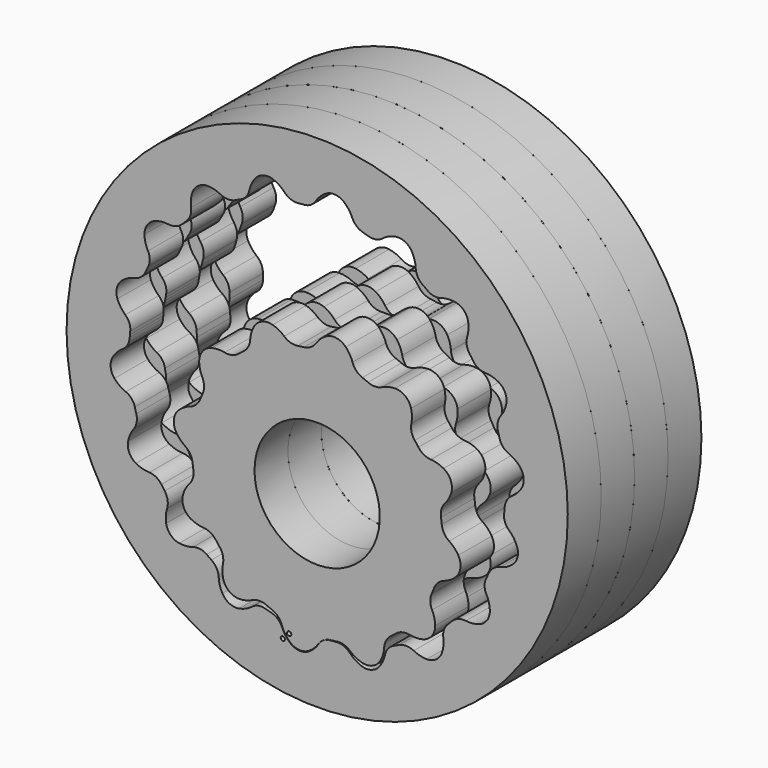
from build123d import *

# Parameters (mm, degrees)
F0_R      = 9.525
F0_R_2    = 0.3175
F1_DEPTH  = 6.35
F0_R_3    = 38.1
F2_DEPTH  = 6.35
F3_R      = 2.54
F4_R      = 2.4892
F5_R      = 2.54
F6_R      = 2.286
F7_R      = 2.413
F9_ANGLE  = 0.02
F11_ANGLE = 7.5
F12_ANGLE = 4.9999
F14_ANGLE = 180
F15_ANGLE = 7.5
F16_ANGLE = 4.9999


with BuildPart() as f1:
    # F0 (on Front) → F1 (new body)
    with BuildSketch(Plane.XZ):
        with BuildLine():
            ThreePointArc((18.7854166667, -3.1639564883), (18.9837389297, -1.5875), (19.05, 0))
            ThreePointArc((19.05, 0), (18.9837389297, 1.5875), (18.7854166667, 3.1639564883))
            ThreePointArc((18.7854166667, 3.1639564883), (18.4008869908, 4.9305028092), (17.8506262981, 6.652641638))
            ThreePointArc((17.8506262981, 6.652641638), (16.4977839421, 9.525), (14.6866698099, 12.1327750287))
            ThreePointArc((14.6866698099, 12.1327750287), (13.4703841816, 13.4703841816), (12.1327750287, 14.6866698099))
            ThreePointArc((12.1327750287, 14.6866698099), (9.525, 16.4977839421), (6.652641638, 17.8506262981))
            ThreePointArc((6.652641638, 17.8506262981), (4.9305028092, 18.4008869908), (3.1639564883, 18.7854166667))
            ThreePointArc((3.1639564883, 18.7854166667), (0, 19.05), (-3.1639564883, 18.7854166667))
            ThreePointArc((-3.1639564883, 18.7854166667), (-4.9305028092, 18.4008869908), (-6.652641638, 17.8506262981))
            ThreePointArc((-6.652641638, 17.8506262981), (-9.525, 16.4977839421), (-12.1327750287, 14.6866698099))
            ThreePointArc((-12.1327750287, 14.6866698099), (-13.4703841816, 13.4703841816), (-14.6866698099, 12.1327750287))
            ThreePointArc((-14.6866698099, 12.1327750287), (-16.4977839421, 9.525), (-17.8506262981, 6.652641638))
            ThreePointArc((-17.8506262981, 6.652641638), (-18.4008869908, 4.9305028092), (-18.7854166667, 3.1639564883))
            ThreePointArc((-18.7854166667, 3.1639564883), (-19.05, 0), (-18.7854166667, -3.1639564883))
            ThreePointArc((-18.7854166667, -3.1639564883), (-18.4008869908, -4.9305028092), (-17.8506262981, -6.652641638))
            ThreePointArc((-17.8506262981, -6.652641638), (-16.4977839421, -9.525), (-14.6866698099, -12.1327750287))
            ThreePointArc((-14.6866698099, -12.1327750287), (-13.4703841816, -13.4703841816), (-12.1327750287, -14.6866698099))
            ThreePointArc((-12.1327750287, -14.6866698099), (-9.525, -16.4977839421), (-6.652641638, -17.8506262981))
            ThreePointArc((-6.652641638, -17.8506262981), (-4.9305028092, -18.4008869908), (-3.1639564883, -18.7854166667))
            ThreePointArc((-3.1639564883, -18.7854166667), (0, -19.05), (3.1639564883, -18.7854166667))
            ThreePointArc((3.1639564883, -18.7854166667), (4.9305028092, -18.4008869908), (6.652641638, -17.8506262981))
            ThreePointArc((6.652641638, -17.8506262981), (9.525, -16.4977839421), (12.1327750287, -14.6866698099))
            ThreePointArc((12.1327750287, -14.6866698099), (13.4703841816, -13.4703841816), (14.6866698099, -12.1327750287))
            ThreePointArc((14.6866698099, -12.1327750287), (16.4977839421, -9.525), (17.8506262981, -6.652641638))
            ThreePointArc((17.8506262981, -6.652641638), (18.4008869908, -4.9305028092), (18.7854166667, -3.1639564883))
        make_face()
        Circle(F0_R, mode=Mode.SUBTRACT)
        with BuildLine():
            ThreePointArc((-3.1639564883, 18.7854166667), (0, 19.05), (3.1639564883, 18.7854166667))
            ThreePointArc((3.1639564883, 18.7854166667), (2.0640323089, 20.9486335794), (0, 22.225))
            ThreePointArc((0, 22.225), (-2.0640323089, 20.9486335794), (-3.1639564883, 18.7854166667))
        make_face()
        with BuildLine():
            ThreePointArc((-12.1327750287, 14.6866698099), (-9.525, 16.4977839421), (-6.652641638, 17.8506262981))
            ThreePointArc((-6.652641638, 17.8506262981), (-8.686812376, 19.1740650088), (-11.1125, 19.2474145991))
            ThreePointArc((-11.1125, 19.2474145991), (-12.2618212034, 17.1100326999), (-12.1327750287, 14.6866698099))
        make_face()
        with BuildLine():
            ThreePointArc((-17.8506262981, 6.652641638), (-16.4977839421, 9.525), (-14.6866698099, 12.1327750287))
            ThreePointArc((-14.6866698099, 12.1327750287), (-17.1100326999, 12.2618212034), (-19.2474145991, 11.1125))
            ThreePointArc((-19.2474145991, 11.1125), (-19.1740650088, 8.686812376), (-17.8506262981, 6.652641638))
        make_face()
        with BuildLine():
            ThreePointArc((-18.7854166667, -3.1639564883), (-19.05, 0), (-18.7854166667, 3.1639564883))
            ThreePointArc((-18.7854166667, 3.1639564883), (-20.9486335794, 2.0640323089), (-22.225, 0))
            ThreePointArc((-22.225, 0), (-20.9486335794, -2.0640323089), (-18.7854166667, -3.1639564883))
        make_face()
        with BuildLine():
            ThreePointArc((-19.2474145991, -11.1125), (-17.1100326999, -12.2618212034), (-14.6866698099, -12.1327750287))
            ThreePointArc((-14.6866698099, -12.1327750287), (-16.4977839421, -9.525), (-17.8506262981, -6.652641638))
            ThreePointArc((-17.8506262981, -6.652641638), (-19.1740650088, -8.686812376), (-19.2474145991, -11.1125))
        make_face()
        with BuildLine():
            ThreePointArc((6.652641638, 17.8506262981), (9.525, 16.4977839421), (12.1327750287, 14.6866698099))
            ThreePointArc((12.1327750287, 14.6866698099), (12.2618212034, 17.1100326999), (11.1125, 19.2474145991))
            ThreePointArc((11.1125, 19.2474145991), (8.686812376, 19.1740650088), (6.652641638, 17.8506262981))
        make_face()
        with BuildLine():
            ThreePointArc((14.6866698099, 12.1327750287), (16.4977839421, 9.525), (17.8506262981, 6.652641638))
            ThreePointArc((17.8506262981, 6.652641638), (19.1740650088, 8.686812376), (19.2474145991, 11.1125))
            ThreePointArc((19.2474145991, 11.1125), (17.1100326999, 12.2618212034), (14.6866698099, 12.1327750287))
        make_face()
        with BuildLine():
            ThreePointArc((18.7854166667, 3.1639564883), (18.9837389297, 1.5875), (19.05, 0))
            ThreePointArc((19.05, 0), (18.9837389297, -1.5875), (18.7854166667, -3.1639564883))
            ThreePointArc((18.7854166667, -3.1639564883), (20.9486335794, -2.0640323089), (22.225, 0))
            ThreePointArc((22.225, 0), (20.9486335794, 2.0640323089), (18.7854166667, 3.1639564883))
        make_face()
        with BuildLine():
            ThreePointArc((19.2474145991, -11.1125), (19.1740650088, -8.686812376), (17.8506262981, -6.652641638))
            ThreePointArc((17.8506262981, -6.652641638), (16.4977839421, -9.525), (14.6866698099, -12.1327750287))
            ThreePointArc((14.6866698099, -12.1327750287), (17.1100326999, -12.2618212034), (19.2474145991, -11.1125))
        make_face()
        with BuildLine():
            ThreePointArc((-11.1125, -19.2474145991), (-8.686812376, -19.1740650088), (-6.652641638, -17.8506262981))
            ThreePointArc((-6.652641638, -17.8506262981), (-9.525, -16.4977839421), (-12.1327750287, -14.6866698099))
            ThreePointArc((-12.1327750287, -14.6866698099), (-12.2618212034, -17.1100326999), (-11.1125, -19.2474145991))
        make_face()
        with BuildLine():
            ThreePointArc((0, -22.225), (2.0640323089, -20.9486335794), (3.1639564883, -18.7854166667))
            ThreePointArc((3.1639564883, -18.7854166667), (0, -19.05), (-3.1639564883, -18.7854166667))
            ThreePointArc((-3.1639564883, -18.7854166667), (-2.0640323089, -20.9486335794), (0, -22.225))
        make_face()
        with Locations((1.5819782441, -20.5052083333)):
            Circle(F0_R_2, mode=Mode.SUBTRACT)
        with BuildLine():
            ThreePointArc((11.1125, -19.2474145991), (12.2618212034, -17.1100326999), (12.1327750287, -14.6866698099))
            ThreePointArc((12.1327750287, -14.6866698099), (9.525, -16.4977839421), (6.652641638, -17.8506262981))
            ThreePointArc((6.652641638, -17.8506262981), (8.686812376, -19.1740650088), (11.1125, -19.2474145991))
        make_face()
    extrude(amount=-F1_DEPTH)

    # F3
    f3_edges = [f1.edges().sort_by_distance(p)[0] for p in [
        (-3.163956, 3.175, -18.785417),
        (3.163956, 3.175, -18.785417),
        (6.652642, 3.175, -17.850626),
        (-6.652642, 3.175, -17.850626),
        (-12.132775, 3.175, -14.68667),
        (-14.68667, 3.175, -12.132775),
        (12.132775, 3.175, -14.68667),
        (14.68667, 3.175, -12.132775),
        (17.850626, 3.175, -6.652642),
        (-17.850626, 3.175, -6.652642),
        (-18.785417, 3.175, -3.163956),
        (-18.785417, 3.175, 3.163956),
        (-17.850626, 3.175, 6.652642),
        (-14.68667, 3.175, 12.132775),
        (-12.132775, 3.175, 14.68667),
        (-6.652642, 3.175, 17.850626),
        (-3.163956, 3.175, 18.785417),
        (3.163956, 3.175, 18.785417),
        (6.652642, 3.175, 17.850626),
        (12.132775, 3.175, 14.68667),
        (14.68667, 3.175, 12.132775),
        (17.850626, 3.175, 6.652642),
        (18.785417, 3.175, 3.163956),
        (18.785417, 3.175, -3.163956),
    ]]
    fillet(f3_edges, radius=F3_R)

    # F4
    f4_edges = [f1.edges().sort_by_distance(p)[0] for p in [
        (0, 3.175, -22.225),
        (11.1125, 3.175, -19.247415),
        (-11.1125, 3.175, -19.247415),
        (-19.247415, 3.175, -11.1125),
        (19.247415, 3.175, -11.1125),
        (22.225, 3.175, 0),
        (-22.225, 3.175, 0),
        (-19.247415, 3.175, 11.1125),
        (-11.1125, 3.175, 19.247415),
        (0, 3.175, 22.225),
        (11.1125, 3.175, 19.247415),
        (19.247415, 3.175, 11.1125),
    ]]
    fillet(f4_edges, radius=F4_R)


with BuildPart() as f2:
    # F0 (on Front) → F2 (new body)
    with BuildSketch(Plane.XZ):
        Circle(F0_R_3)
        with Locations((2.5347402211, -30.9479771842)):
            Circle(F0_R_2, mode=Mode.SUBTRACT)
        with BuildLine():
            ThreePointArc((28.517262004, 1.8155970902), (28.5605618534, 0.9082574621), (28.575, 0))
            ThreePointArc((28.575, 0), (28.5605618534, -0.9082574621), (28.517262004, -1.8155970902))
            ThreePointArc((28.517262004, -1.8155970902), (30.3985169788, -3.2859843886), (31.2615712993, -5.5122584794))
            ThreePointArc((31.2615712993, -5.5122584794), (29.6891349394, -7.309089852), (27.4184314472, -8.0473748499))
            ThreePointArc((27.4184314472, -8.0473748499), (26.851716639, -9.7732255955), (26.1764898932, -11.4595812258))
            ThreePointArc((26.1764898932, -11.4595812258), (27.4413892362, -13.484720416), (27.490964429, -15.8719157133))
            ThreePointArc((27.490964429, -15.8719157133), (25.3988050613, -17.0225799857), (23.0125334049, -16.9397146165))
            ThreePointArc((23.0125334049, -16.9397146165), (21.8897199621, -18.3676559468), (20.6784467774, -19.7213707403))
            ThreePointArc((20.6784467774, -19.7213707403), (21.17442496, -22.0570001479), (20.4045415251, -24.3171856677))
            ThreePointArc((20.4045415251, -24.3171856677), (18.0450044464, -24.6828957467), (15.8309842052, -23.7888747968))
            ThreePointArc((15.8309842052, -23.7888747968), (14.2875, -24.7466759131), (12.6862777989, -25.604471887))
            ThreePointArc((12.6862777989, -25.604471887), (12.3535125324, -27.9688801353), (10.8570297743, -29.8294441471))
            ThreePointArc((10.8570297743, -29.8294441471), (8.5147099793, -29.3660899998), (6.7399846698, -27.7687455902))
            ThreePointArc((6.7399846698, -27.7687455902), (4.9619966768, -28.1408815423), (3.1639564883, -28.3992958423))
            ThreePointArc((3.1639564883, -28.3992958423), (2.0425841749, -30.5073004017), (0, -31.7438314267))
            ThreePointArc((0, -31.7438314267), (-2.0425841749, -30.5073004017), (-3.1639564883, -28.3992958423))
            ThreePointArc((-3.1639564883, -28.3992958423), (-4.9619966768, -28.1408815423), (-6.7399846698, -27.7687455902))
            ThreePointArc((-6.7399846698, -27.7687455902), (-8.5147099793, -29.3660899998), (-10.8570297743, -29.8294441471))
            ThreePointArc((-10.8570297743, -29.8294441471), (-12.3535125324, -27.9688801353), (-12.6862777989, -25.604471887))
            ThreePointArc((-12.6862777989, -25.604471887), (-14.2875, -24.7466759131), (-15.8309842052, -23.7888747968))
            ThreePointArc((-15.8309842052, -23.7888747968), (-18.0450044464, -24.6828957467), (-20.4045415251, -24.3171856677))
            ThreePointArc((-20.4045415251, -24.3171856677), (-21.17442496, -22.0570001479), (-20.6784467774, -19.7213707403))
            ThreePointArc((-20.6784467774, -19.7213707403), (-21.8897199621, -18.3676559468), (-23.0125334049, -16.9397146165))
            ThreePointArc((-23.0125334049, -16.9397146165), (-25.3988050613, -17.0225799857), (-27.490964429, -15.8719157133))
            ThreePointArc((-27.490964429, -15.8719157133), (-27.4413892362, -13.484720416), (-26.1764898932, -11.4595812258))
            ThreePointArc((-26.1764898932, -11.4595812258), (-26.851716639, -9.7732255955), (-27.4184314472, -8.0473748499))
            ThreePointArc((-27.4184314472, -8.0473748499), (-29.6891349394, -7.309089852), (-31.2615712993, -5.5122584794))
            ThreePointArc((-31.2615712993, -5.5122584794), (-30.3985169788, -3.2859843886), (-28.517262004, -1.8155970902))
            ThreePointArc((-28.517262004, -1.8155970902), (-28.575, 0), (-28.517262004, 1.8155970902))
            ThreePointArc((-28.517262004, 1.8155970902), (-30.3985169788, 3.2859843886), (-31.2615712993, 5.5122584794))
            ThreePointArc((-31.2615712993, 5.5122584794), (-29.6891349394, 7.309089852), (-27.4184314472, 8.0473748499))
            ThreePointArc((-27.4184314472, 8.0473748499), (-26.851716639, 9.7732255955), (-26.1764898932, 11.4595812258))
            ThreePointArc((-26.1764898932, 11.4595812258), (-27.4413892362, 13.484720416), (-27.490964429, 15.8719157133))
            ThreePointArc((-27.490964429, 15.8719157133), (-25.3988050613, 17.0225799857), (-23.0125334049, 16.9397146165))
            ThreePointArc((-23.0125334049, 16.9397146165), (-21.8897199621, 18.3676559468), (-20.6784467774, 19.7213707403))
            ThreePointArc((-20.6784467774, 19.7213707403), (-21.17442496, 22.0570001479), (-20.4045415251, 24.3171856677))
            ThreePointArc((-20.4045415251, 24.3171856677), (-18.0450044464, 24.6828957467), (-15.8309842052, 23.7888747968))
            ThreePointArc((-15.8309842052, 23.7888747968), (-14.2875, 24.7466759131), (-12.6862777989, 25.604471887))
            ThreePointArc((-12.6862777989, 25.604471887), (-12.3535125324, 27.9688801353), (-10.8570297743, 29.8294441471))
            ThreePointArc((-10.8570297743, 29.8294441471), (-8.5147099793, 29.3660899998), (-6.7399846698, 27.7687455902))
            ThreePointArc((-6.7399846698, 27.7687455902), (-4.9619966768, 28.1408815423), (-3.1639564883, 28.3992958423))
            ThreePointArc((-3.1639564883, 28.3992958423), (-2.0425841749, 30.5073004017), (0, 31.7438314267))
            ThreePointArc((0, 31.7438314267), (2.0425841749, 30.5073004017), (3.1639564883, 28.3992958423))
            ThreePointArc((3.1639564883, 28.3992958423), (4.9619966768, 28.1408815423), (6.7399846698, 27.7687455902))
            ThreePointArc((6.7399846698, 27.7687455902), (8.5147099793, 29.3660899998), (10.8570297743, 29.8294441471))
            ThreePointArc((10.8570297743, 29.8294441471), (12.3535125324, 27.9688801353), (12.6862777989, 25.604471887))
            ThreePointArc((12.6862777989, 25.604471887), (14.2875, 24.7466759131), (15.8309842052, 23.7888747968))
            ThreePointArc((15.8309842052, 23.7888747968), (18.0450044464, 24.6828957467), (20.4045415251, 24.3171856677))
            ThreePointArc((20.4045415251, 24.3171856677), (21.17442496, 22.0570001479), (20.6784467774, 19.7213707403))
            ThreePointArc((20.6784467774, 19.7213707403), (21.8897199621, 18.3676559468), (23.0125334049, 16.9397146165))
            ThreePointArc((23.0125334049, 16.9397146165), (25.3988050613, 17.0225799857), (27.490964429, 15.8719157133))
            ThreePointArc((27.490964429, 15.8719157133), (27.4413892362, 13.484720416), (26.1764898932, 11.4595812258))
            ThreePointArc((26.1764898932, 11.4595812258), (26.851716639, 9.7732255955), (27.4184314472, 8.0473748499))
            ThreePointArc((27.4184314472, 8.0473748499), (29.6891349394, 7.309089852), (31.2615712993, 5.5122584794))
            ThreePointArc((31.2615712993, 5.5122584794), (30.3985169788, 3.2859843886), (28.517262004, 1.8155970902))
        make_face(mode=Mode.SUBTRACT)
    extrude(amount=-F2_DEPTH)

    # F5
    f5_edges = [f2.edges().sort_by_distance(p)[0] for p in [
        (3.163956, 3.175, -28.399296),
        (12.686278, 3.175, -25.604472),
        (20.678447, 3.175, -19.721371),
        (-6.739985, 3.175, -27.768746),
        (-15.830984, 3.175, -23.788875),
        (-23.012533, 3.175, -16.939715),
        (-27.418431, 3.175, -8.047375),
        (26.17649, 3.175, -11.459581),
        (28.517262, 3.175, -1.815597),
        (27.418431, 3.175, 8.047375),
        (23.012533, 3.175, 16.939715),
        (-28.517262, 3.175, 1.815597),
        (-26.17649, 3.175, 11.459581),
        (-20.678447, 3.175, 19.721371),
        (-12.686278, 3.175, 25.604472),
        (-3.163956, 3.175, 28.399296),
        (6.739985, 3.175, 27.768746),
        (15.830984, 3.175, 23.788875),
    ]]
    fillet(f5_edges, radius=F5_R)

    # F6
    f6_edges = [f2.edges().sort_by_distance(p)[0] for p in [
        (-3.163956, 3.175, -28.399296),
        (6.739985, 3.175, -27.768746),
        (-12.686278, 3.175, -25.604472),
        (-20.678447, 3.175, -19.721371),
        (15.830984, 3.175, -23.788875),
        (23.012533, 3.175, -16.939715),
        (-26.17649, 3.175, -11.459581),
        (-28.517262, 3.175, -1.815597),
        (27.418431, 3.175, -8.047375),
        (28.517262, 3.175, 1.815597),
        (26.17649, 3.175, 11.459581),
        (20.678447, 3.175, 19.721371),
        (12.686278, 3.175, 25.604472),
        (3.163956, 3.175, 28.399296),
        (-6.739985, 3.175, 27.768746),
        (-15.830984, 3.175, 23.788875),
        (-23.012533, 3.175, 16.939715),
        (-27.418431, 3.175, 8.047375),
    ]]
    fillet(f6_edges, radius=F6_R)

    # F7
    f7_edges = [f2.edges().sort_by_distance(p)[0] for p in [
        (0, 3.175, -31.743831),
        (10.85703, 3.175, -29.829444),
        (20.404542, 3.175, -24.317186),
        (27.490964, 3.175, -15.871916),
        (-10.85703, 3.175, -29.829444),
        (-20.404542, 3.175, -24.317186),
        (-27.490964, 3.175, -15.871916),
        (-31.261571, 3.175, -5.512258),
        (-31.261571, 3.175, 5.512258),
        (31.261571, 3.175, -5.512258),
        (31.261571, 3.175, 5.512258),
        (27.490964, 3.175, 15.871916),
        (-27.490964, 3.175, 15.871916),
        (-20.404542, 3.175, 24.317186),
        (-10.85703, 3.175, 29.829444),
        (0, 3.175, 31.743831),
        (20.404542, 3.175, 24.317186),
        (10.85703, 3.175, 29.829444),
    ]]
    fillet(f7_edges, radius=F7_R)


with BuildPart() as f1_1:
    # F8: moved
    add(f1.part.moved(Location((0, 0, -9.5123))))


with BuildPart() as f1_2:
    # F9: moved
    add(f1_1.part.rotate(Axis((0, 0, -9.5123), (0, -1, 0)), F9_ANGLE))


with BuildPart() as f10_1:
    # F10: copy of F1
    add(f1_2.part.moved(Location((0, 6.35, 0))))


with BuildPart() as f10_2:
    # F10: copy of F2
    add(f2.part.moved(Location((0, 6.35, 0))))


with BuildPart() as f1_3:
    # F11: moved
    add(f1_2.part.rotate(Axis((0, 0, -9.5123), (0, -1, 0)), F11_ANGLE))


with BuildPart() as f2_1:
    # F12: moved
    add(f2.part.rotate(Axis((0, 0, 0), (0, -1, 0)), F12_ANGLE))


with BuildPart() as f14_1:
    # F14: copy of F10_1
    add(f10_1.part.rotate(Axis((0, 0, 0), (0, 0, 1)), F14_ANGLE))


with BuildPart() as f14_2:
    # F14: copy of F1
    add(f1_3.part.rotate(Axis((0, 0, 0), (0, 0, 1)), F14_ANGLE))


with BuildPart() as f14_3:
    # F14: copy of F10_2
    add(f10_2.part.rotate(Axis((0, 0, 0), (0, 0, 1)), F14_ANGLE))


with BuildPart() as f14_4:
    # F14: copy of F2
    add(f2_1.part.rotate(Axis((0, 0, 0), (0, 0, 1)), F14_ANGLE))


with BuildPart() as f14_2_1:
    # F15: moved
    add(f14_2.part.rotate(Axis((0, -12.7, -9.5123), (0, 1, 0)), F15_ANGLE))


with BuildPart() as f14_1_1:
    # F15: moved
    add(f14_1.part.rotate(Axis((0, -12.7, -9.5123), (0, 1, 0)), F15_ANGLE))


with BuildPart() as f14_4_1:
    # F16: moved
    add(f14_4.part.rotate(Axis((0, -12.7, 0), (0, 1, 0)), F16_ANGLE))


with BuildPart() as f14_3_1:
    # F16: moved
    add(f14_3.part.rotate(Axis((0, -12.7, 0), (0, 1, 0)), F16_ANGLE))


solid = Compound([f10_1.part, f10_2.part, f1_3.part, f2_1.part, f14_2_1.part, f14_1_1.part, f14_4_1.part, f14_3_1.part])
